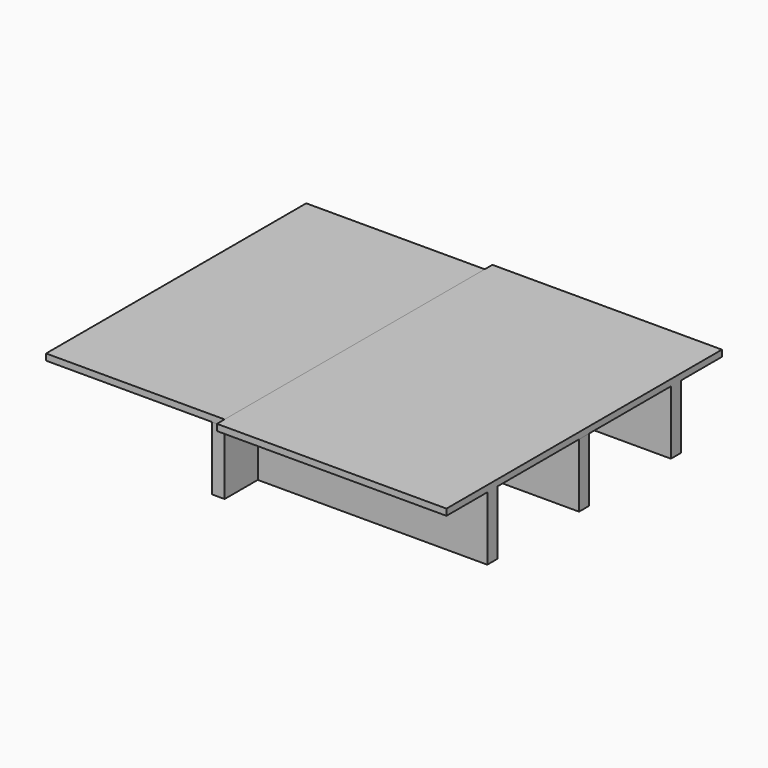
from build123d import *

# Parameters (mm, degrees)
F0_W      = 914.4
F0_H      = 1371.6
F1_DEPTH  = 25.4
F2_W      = 660.4
F2_H      = 1295.4
F3_DEPTH  = 25.4
F4_W      = 914.4
F4_H      = 254
F5_DEPTH  = 25.4
F6_W      = 914.4
F6_H      = 50.8
F7_DEPTH  = 254
F9_W      = 165.1
F9_H      = 254
F9_W_2    = 863.6
F10_DEPTH = 50.8
F11_W     = 1295.4
F11_H     = 25.4
F12_DEPTH = 50.8
F13_W     = 711.2
F13_H     = 1295.4
F14_DEPTH = 25.4


with BuildPart() as f1:
    # F0 (on Top) → F1 (new body)
    with BuildSketch(Plane.XY):
        Rectangle(F0_W, F0_H)
    extrude(amount=F1_DEPTH)

    # F6 (on face) → F7 (join)
    with BuildSketch(Plane(origin=(0, 0, 0), x_dir=(1, 0, 0), z_dir=(0, 0, -1))):
        with Locations((0, 457.2)):
            Rectangle(F6_W, F6_H)
        with Locations((0, -457.2)):
            Rectangle(F6_W, F6_H)
    extrude(amount=F7_DEPTH)


with BuildPart() as f3:
    # F2 (on Top) → F3 (new body)
    with BuildSketch(Plane.XY):
        with Locations((-993.5793445587, 28.9456365585)):
            Rectangle(F2_W, F2_H)
    extrude(amount=F3_DEPTH)


with BuildPart() as f5:
    # F4 (on Front) → F5 (new body, symmetric)
    with BuildSketch(Plane.XZ):
        with Locations((-0.2912971497, -127)):
            Rectangle(F4_W, F4_H)
    extrude(amount=F5_DEPTH, both=True)


with BuildPart() as f10:
    # F9 (on face) → F10 (new body)
    with BuildSketch(Plane(origin=(-457.2, 0, 0), x_dir=(0, -1, 0), z_dir=(-1, 0, 0))):
        Polygon((647.7, 25.4), (-647.7, 25.4), (-647.7, 0), (-482.6, 0), (-482.6, -254), (-431.8, -254), (-431.8, 0), (431.8, 0), (431.8, -254), (482.6, -254), (482.6, 0), (647.7, 0), align=None)
        Polygon((-482.6, 0), (-647.7, 0), (-647.7, -174.1451999916), (-647.7, -254), (-482.6, -254), align=None)
        with Locations((565.15, -127)):
            Rectangle(F9_W, F9_H)
        with Locations((0, -127)):
            Rectangle(F9_W_2, F9_H)
    extrude(amount=F10_DEPTH)

    # F11 (on face) → F12 (cut)
    with BuildSketch(Plane(origin=(-508, 0, 0), x_dir=(0, -1, 0), z_dir=(-1, 0, 0))):
        with Locations((0, 12.7)):
            Rectangle(F11_W, F11_H)
    extrude(amount=-F12_DEPTH, mode=Mode.SUBTRACT)


with BuildPart() as f14:
    # F13 (on face) → F14 (new body)
    with BuildSketch(Plane.XY):
        with Locations((-812.8, 0)):
            Rectangle(F13_W, F13_H)
    extrude(amount=F14_DEPTH)


solid = Compound([f1.part, f5.part, f10.part, f14.part])
